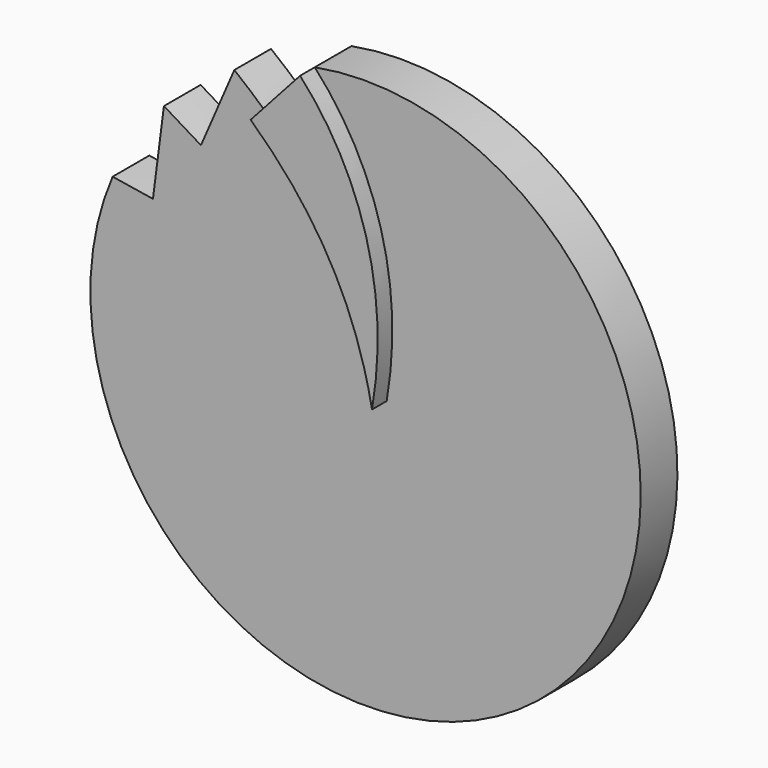
from build123d import *

# Parameters (mm, degrees)
F0_R     = 30
F1_DEPTH = 5
F4_DEPTH = 5
F5_DEPTH = 5
F6_DEPTH = 5
F7_DEPTH = 2


with BuildPart() as f1:
    # F0 (on Front) → F1 (new body)
    with BuildSketch(Plane.XZ):
        Circle(F0_R)
    extrude(amount=F1_DEPTH)

    # F3 (on face) → F4 (cut)
    with BuildSketch(Plane.XZ.offset(5)):
        with BuildLine():
            Line((-10.9299741999, 23.5023200512), (-5.5388955, 29.4842438709))
            ThreePointArc((-5.5388955, 29.4842438709), (-10.0449779303, 28.2683288926), (-14.3079358656, 26.3682189627))
            add(Edge.make_bspline(
                [(-14.3079358656, 26.3682189627), (-13.1550391421, 25.4607855158), (-12.0252922437, 24.5080470289), (-10.9299741999, 23.5023200512)],
                knots=[0, 0, 0, 0, 4.6870131966, 4.6870131966, 4.6870131966, 4.6870131966], degree=3))
        make_face()
    extrude(amount=-F4_DEPTH, mode=Mode.SUBTRACT)

    # F3 (on face) → F5 (cut)
    with BuildSketch(Plane.XZ.offset(5)):
        with BuildLine():
            Line((-17.9465766996, 17.9648566991), (-14.3079358656, 26.3682189627))
            ThreePointArc((-14.3079358656, 26.3682189627), (-18.3884401049, 23.7036974016), (-21.9836899596, 20.4136565995))
            add(Edge.make_bspline(
                [(-21.9836899596, 20.4136565995), (-20.642975191, 19.610865703), (-19.293517456, 18.7987052228), (-17.9465766996, 17.9648566991)],
                knots=[0, 0, 0, 0, 4.8486235733, 4.8486235733, 4.8486235733, 4.8486235733], degree=3))
        make_face()
    extrude(amount=-F5_DEPTH, mode=Mode.SUBTRACT)

    # F3 (on face) → F6 (cut)
    with BuildSketch(Plane.XZ.offset(5)):
        with BuildLine():
            Line((-23.1792298082, 11.114937143), (-21.9836899596, 20.4136565995))
            ThreePointArc((-21.9836899596, 20.4136565995), (-25.1493367192, 16.3557593094), (-27.5748147519, 11.8164965789))
            add(Edge.make_bspline(
                [(-27.5748147519, 11.8164965789), (-26.208679714, 11.6220681724), (-24.7320616466, 11.3922656282), (-23.1792298082, 11.114937143)],
                knots=[0, 0, 0, 0, 5.1239362549, 5.1239362549, 5.1239362549, 5.1239362549], degree=3))
        make_face()
    extrude(amount=-F6_DEPTH, mode=Mode.SUBTRACT)

    # F3 (on face) → F7 (join)
    with BuildSketch(Plane.XZ.offset(5)):
        with BuildLine():
            add(Edge.make_bspline(
                [(-5.5388955, 29.4842438709), (0, 23.5023200512), (4.6262064465, 13.365700841), (2.3032309004, 0)],
                knots=[0, 0, 0, 0, 30.5093359993, 30.5093359993, 30.5093359993, 30.5093359993], degree=3))
            Line((-5.5388955, 29.4842438709), (-10.9299741999, 23.5023200512))
            add(Edge.make_bspline(
                [(-10.9299741999, 23.5023200512), (-4.7424400597, 17.8208925919), (0.3463986774, 10.4484936531), (2.3032309004, 0)],
                knots=[4.6870131966, 4.6870131966, 4.6870131966, 4.6870131966, 31.1643038201, 31.1643038201, 31.1643038201, 31.1643038201], degree=3))
        make_face()
    extrude(amount=F7_DEPTH)


solid = f1.part
